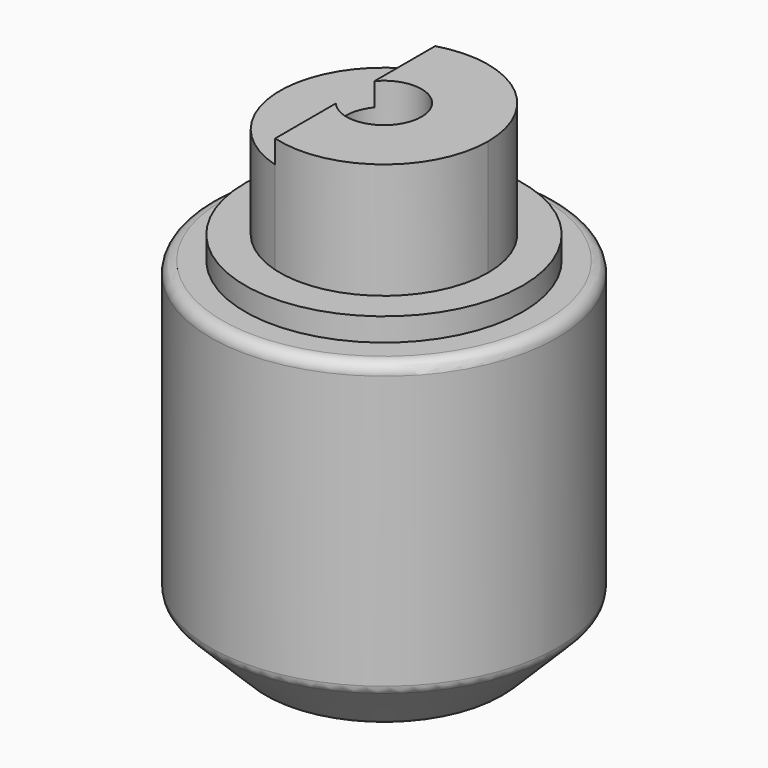
from build123d import *

# Parameters (mm, degrees)
F0_R           = 15
F1_DEPTH       = 30
F2_R           = 12
F3_DEPTH       = 2
F5_DEPTH       = 10
F6_DEPTH       = 8
F7_D           = 6.5
F7_CBORE_D     = 13
F7_CBORE_DEPTH = 15
F8_SIZE        = 5
F9_R           = 1


with BuildPart() as f1:
    # F0 (on Top) → F1 (new body)
    with BuildSketch(Plane.XY):
        Circle(F0_R)
    extrude(amount=F1_DEPTH)

    # F2 (on face) → F3 (join)
    with BuildSketch(Plane.XY.offset(30)):
        Circle(F2_R)
    extrude(amount=F3_DEPTH)

    # F4 (on face) → F5 (join)
    with BuildSketch(Plane.XY.offset(32)):
        with BuildLine():
            ThreePointArc((-2.492736493, -8.6479052248), (5.411347871, -7.1914751073), (9, 0))
            ThreePointArc((9, 0), (5.411347871, 7.1914751073), (-2.492736493, 8.6479052248))
            Line((-2.492736493, 8.6479052248), (-2.492736493, -8.6479052248))
        make_face()
    extrude(amount=F5_DEPTH)

    # F4 (on face) → F6 (join)
    with BuildSketch(Plane.XY.offset(32)):
        with BuildLine():
            Line((-2.492736493, -8.6479052248), (-2.492736493, 8.6479052248))
            ThreePointArc((-2.492736493, 8.6479052248), (-9, 0), (-2.492736493, -8.6479052248))
        make_face()
    extrude(amount=F6_DEPTH)

    # F7 (through all)
    with Locations(Plane(origin=(0, 0, 0), x_dir=(1, 0, 0), z_dir=(0, 0, -1))):
        with Locations((0, 0)):
            CounterBoreHole(F7_D / 2, F7_CBORE_D / 2, F7_CBORE_DEPTH)

    # F8
    f8_edges = [f1.edges().sort_by_distance(p)[0] for p in [
        (-15, 0, 0),
    ]]
    chamfer(f8_edges, length=F8_SIZE)

    # F9
    f9_edges = [f1.edges().sort_by_distance(p)[0] for p in [
        (-15, 0, 30),
        (-10, 0, 0),
        (-15, 0, 5),
        (-6.5, 0, 0),
    ]]
    fillet(f9_edges, radius=F9_R)


solid = f1.part
